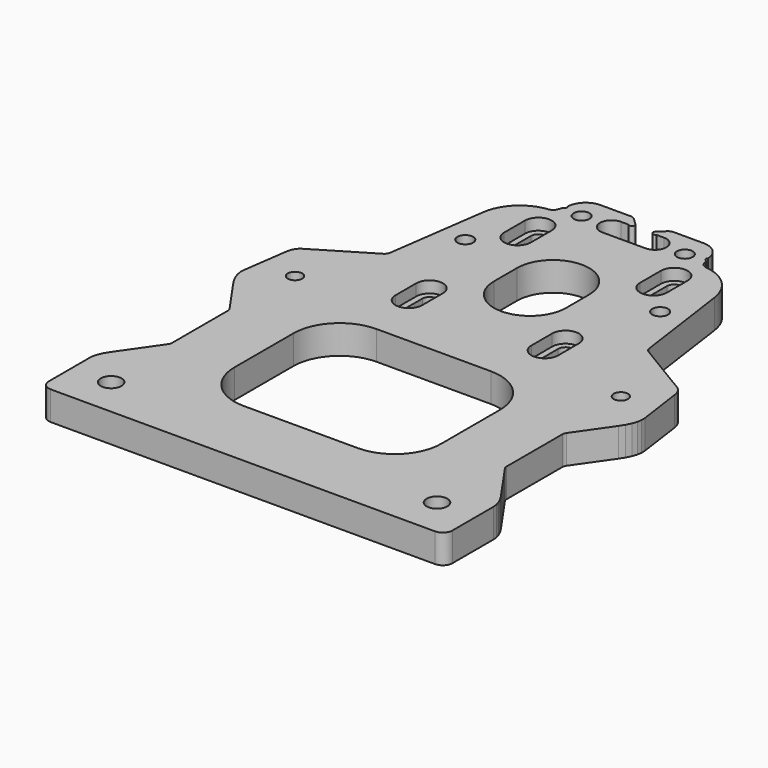
from build123d import *

# Parameters (mm, degrees)
F0_R     = 4.1
F0_R_2   = 2.725
F0_R_3   = 2.5
F0_R_4   = 3.6
F1_DEPTH = 10
F2_DEPTH = 6
F3_DEPTH = 4


# Not quite as in the source:
# - ends of sketch curves that miss each other by under 0.0002 mm in the source are joined


with BuildPart() as f1:
    # F0 (on Top) → F1 (new body)
    with BuildSketch(Plane.XY):
        with BuildLine():
            ThreePointArc((-70, -85.3407), (-69.01608381, -87.71608381), (-66.6407, -88.7))
            Line((-66.6407, -88.7), (66.64, -88.7))
            ThreePointArc((66.64, -88.7), (69.0158787848, -87.7158787848), (70, -85.34))
            Line((70, -85.34), (70, -67.5895))
            Line((70, -67.5895), (69.865948, -66.201885))
            Line((69.865948, -66.201885), (69.445962, -64.711612))
            Line((69.445962, -64.711612), (68.73318, -63.151071))
            Line((68.73318, -63.151071), (67.734412, -61.538447))
            Line((67.734412, -61.538447), (58.431324, -48.174831))
            ThreePointArc((58.431324, -48.174831), (58.1178035717, -47.5357835753), (58.01, -46.832182))
            Line((58.01, -46.832182), (58.01, -22.760348))
            ThreePointArc((58.01, -22.760348), (58.1179689174, -22.0562197272), (58.4319545741, -21.4167927032))
            Line((58.4319545741, -21.4167927032), (66.783489, -9.432068))
            Line((66.783489, -9.432068), (67.913719, -7.648339))
            Line((67.913719, -7.648339), (68.762828, -5.93532))
            Line((68.762828, -5.93532), (69.316332, -4.305329))
            Line((69.316332, -4.305329), (69.565046, -2.784029))
            Line((69.565046, -2.784029), (69.518711, -1.391715))
            Line((69.518711, -1.391715), (67.309142, 14.330181))
            Line((67.309142, 14.330181), (66.999212, 15.650057))
            Line((66.999212, 15.650057), (66.487155, 16.737863))
            Line((66.487155, 16.737863), (65.781814, 17.619854))
            Line((65.781814, 17.619854), (64.875084, 18.317561))
            Line((64.875084, 18.317561), (46.034788, 29.637953))
            ThreePointArc((46.034788, 29.637953), (45.2854954651, 30.3552438624), (44.917997067, 31.3252390094))
            Line((44.917997067, 31.3252390094), (40.093666, 65.65214))
            ThreePointArc((40.093666, 65.65214), (35.8358190199, 74.0012505725), (27.3375349502, 77.9529685197))
            ThreePointArc((27.3375349502, 77.9529685197), (26.1084756666, 78.4580664195), (25.3498539146, 79.5490309716))
            Line((25.3498539146, 79.5490309716), (24.828406, 81.117409))
            ThreePointArc((24.828406, 81.117409), (24.1173215696, 81.671357459), (24.355163875, 82.5408001437))
            ThreePointArc((24.355163875, 82.5408001437), (22.3679675258, 86.9125704183), (17.910791, 88.7))
            Line((17.910791, 88.7), (7.437437, 88.7))
            ThreePointArc((7.437437, 88.7), (6.5667217917, 88.5327402562), (5.8199517771, 88.0547702349))
            Line((5.8199517771, 88.0547702349), (3.5, 85.8536))
            ThreePointArc((3.5, 85.8536), (3.4660810953, 84.4733300764), (4.8463500657, 84.5072999404))
            Line((4.8463500657, 84.5072999404), (7.5, 84.5073))
            ThreePointArc((7.5, 84.5073), (11.5, 80.5073), (7.5, 76.5073))
            Line((7.5, 76.5073), (-7.5, 76.5073))
            ThreePointArc((-7.5, 76.5073), (-11.5, 80.5073), (-7.5, 84.5073))
            Line((-7.5, 84.5073), (-4.84635, 84.5073))
            ThreePointArc((-4.84635, 84.5073), (-3.4660810953, 84.4733300764), (-3.4999997219, 85.8536003068))
            Line((-3.4999997219, 85.8536003068), (-5.819951, 88.05477))
            ThreePointArc((-5.819951, 88.05477), (-6.5667214548, 88.5327401218), (-7.437437, 88.7))
            Line((-7.437437, 88.7), (-17.91079, 88.7))
            ThreePointArc((-17.91079, 88.7), (-22.3679665258, 86.9125704183), (-24.3551631887, 82.5408000085))
            ThreePointArc((-24.3551631887, 82.5408000085), (-24.1173207269, 81.6713569858), (-24.8284060254, 81.1174093435))
            Line((-24.8284060254, 81.1174093435), (-25.349853, 79.549031))
            ThreePointArc((-25.349853, 79.549031), (-26.1084746666, 78.4580664195), (-27.3375339495, 77.9529685125))
            ThreePointArc((-27.3375339495, 77.9529685125), (-35.8358186118, 74.001250966), (-40.0936657548, 65.6521401061))
            Line((-40.0936657548, 65.6521401061), (-44.917996, 31.325239))
            ThreePointArc((-44.917996, 31.325239), (-45.2854944651, 30.3552438624), (-46.0347868046, 29.6379526747))
            Line((-46.0347868046, 29.6379526747), (-64.875083, 18.317561))
            Line((-64.875083, 18.317561), (-65.764804, 17.636264))
            Line((-65.764804, 17.636264), (-66.464414, 16.773352))
            Line((-66.464414, 16.773352), (-66.99028, 15.673609))
            Line((-66.99028, 15.673609), (-67.30828, 14.330181))
            Line((-67.30828, 14.330181), (-69.517848, -1.391715))
            Line((-69.517848, -1.391715), (-69.564686, -2.784465))
            Line((-69.564686, -2.784465), (-69.316601, -4.307546))
            Line((-69.316601, -4.307546), (-68.763454, -5.938605))
            Line((-68.763454, -5.938605), (-67.915019, -7.650791))
            Line((-67.915019, -7.650791), (-66.786009, -9.432068))
            Line((-66.786009, -9.432068), (-58.427898, -21.419694))
            ThreePointArc((-58.427898, -21.419694), (-58.1136589115, -22.059327239), (-58.0056, -22.763742))
            Line((-58.0056, -22.763742), (-58.0056, -46.834916))
            ThreePointArc((-58.0056, -46.834916), (-58.1134934129, -47.5388038122), (-58.4272664273, -48.1780577023))
            Line((-58.4272664273, -48.1780577023), (-67.733176, -61.538447))
            Line((-67.733176, -61.538447), (-68.732469, -63.151034))
            Line((-68.732469, -63.151034), (-69.445644, -64.711573))
            Line((-69.445644, -64.711573), (-69.865872, -66.201869))
            Line((-69.865872, -66.201869), (-70, -67.5895))
            Line((-70, -67.5895), (-70, -85.3407))
        make_face()
        with Locations((-56.5, -75.18)):
            Circle(F0_R, mode=Mode.SUBTRACT)
        with Locations((56.5, -75.18)):
            Circle(F0_R, mode=Mode.SUBTRACT)
        with BuildLine():
            Line((19.8032, -63.6519), (-19.8032, -63.6519))
            ThreePointArc((-19.8032, -63.6519), (-31.1500010963, -58.9519010963), (-35.85, -47.6051))
            Line((-35.85, -47.6051), (-35.85, -21.9987))
            ThreePointArc((-35.85, -21.9987), (-31.1500010963, -10.6518989037), (-19.8032, -5.9519))
            Line((-19.8032, -5.9519), (19.8032, -5.9519))
            ThreePointArc((19.8032, -5.9519), (31.1500010963, -10.6518989037), (35.85, -21.9987))
            Line((35.85, -21.9987), (35.85, -47.6051))
            ThreePointArc((35.85, -47.6051), (31.1500010963, -58.9519010963), (19.8032, -63.6519))
        make_face(mode=Mode.SUBTRACT)
        with Locations((-56.5, 4.52)):
            Circle(F0_R, mode=Mode.SUBTRACT)
        with BuildLine():
            Line((-28.21, 12.7), (-28.21, 21.7))
            ThreePointArc((-28.21, 21.7), (-23.57, 26.34), (-18.93, 21.7))
            Line((-18.93, 21.7), (-18.93, 12.7))
            ThreePointArc((-18.93, 12.7), (-23.57, 8.06), (-28.21, 12.7))
        make_face(mode=Mode.SUBTRACT)
        with Locations((-33.8, 49.95)):
            Circle(F0_R_2, mode=Mode.SUBTRACT)
        with BuildLine():
            Line((-28.21, 59.84), (-28.21, 68.84))
            ThreePointArc((-28.21, 68.84), (-23.57, 73.48), (-18.93, 68.84))
            Line((-18.93, 68.84), (-18.93, 59.84))
            ThreePointArc((-18.93, 59.84), (-23.57, 55.2), (-28.21, 59.84))
        make_face(mode=Mode.SUBTRACT)
        with Locations((-17.9, 80.5073)):
            Circle(F0_R_2, mode=Mode.SUBTRACT)
        with BuildLine():
            Line((18.93, 12.7), (18.93, 21.7))
            ThreePointArc((18.93, 21.7), (23.57, 26.34), (28.21, 21.7))
            Line((28.21, 21.7), (28.21, 12.7))
            ThreePointArc((28.21, 12.7), (23.57, 8.06), (18.93, 12.7))
        make_face(mode=Mode.SUBTRACT)
        with BuildLine():
            Line((-12.5, 35.77), (-12.5, 45.77))
            ThreePointArc((-12.5, 45.77), (0, 58.27), (12.5, 45.77))
            Line((12.5, 45.77), (12.5, 35.77))
            ThreePointArc((12.5, 35.77), (0, 23.27), (-12.5, 35.77))
        make_face(mode=Mode.SUBTRACT)
        with Locations((56.5, 4.52)):
            Circle(F0_R, mode=Mode.SUBTRACT)
        with Locations((33.8, 49.95)):
            Circle(F0_R_2, mode=Mode.SUBTRACT)
        with BuildLine():
            Line((18.93, 59.84), (18.93, 68.84))
            ThreePointArc((18.93, 68.84), (23.57, 73.48), (28.21, 68.84))
            Line((28.21, 68.84), (28.21, 59.84))
            ThreePointArc((28.21, 59.84), (23.57, 55.2), (18.93, 59.84))
        make_face(mode=Mode.SUBTRACT)
        with Locations((17.9, 80.5073)):
            Circle(F0_R_2, mode=Mode.SUBTRACT)
        with Locations((-56.5, 4.52)):
            Circle(F0_R)
        with Locations((-56.5, 4.52)):
            Circle(F0_R_3, mode=Mode.SUBTRACT)
        with Locations((56.5, 4.52)):
            Circle(F0_R)
        with Locations((56.5, 4.52)):
            Circle(F0_R_3, mode=Mode.SUBTRACT)
        with Locations((56.5, -75.18)):
            Circle(F0_R)
        with Locations((56.5, -75.18)):
            Circle(F0_R_4, mode=Mode.SUBTRACT)
        with Locations((-56.5, -75.18)):
            Circle(F0_R)
        with Locations((-56.5, -75.18)):
            Circle(F0_R_4, mode=Mode.SUBTRACT)
    extrude(amount=F1_DEPTH)

    # F0 (on Top) → F2 (join)
    with BuildSketch(Plane.XY):
        with BuildLine():
            ThreePointArc((-18.93, 21.7), (-23.57, 26.34), (-28.21, 21.7))
            Line((-28.21, 21.7), (-28.21, 12.7))
            ThreePointArc((-28.21, 12.7), (-23.57, 8.06), (-18.93, 12.7))
            Line((-18.93, 12.7), (-18.93, 21.7))
        make_face()
        with BuildLine():
            Line((-26.11, 12.7), (-26.11, 21.7))
            ThreePointArc((-26.11, 21.7), (-23.57, 24.24), (-21.03, 21.7))
            Line((-21.03, 21.7), (-21.03, 12.7))
            ThreePointArc((-21.03, 12.7), (-23.57, 10.16), (-26.11, 12.7))
        make_face(mode=Mode.SUBTRACT)
        with BuildLine():
            ThreePointArc((-18.93, 68.84), (-23.57, 73.48), (-28.21, 68.84))
            Line((-28.21, 68.84), (-28.21, 59.84))
            ThreePointArc((-28.21, 59.84), (-23.57, 55.2), (-18.93, 59.84))
            Line((-18.93, 59.84), (-18.93, 68.84))
        make_face()
        with BuildLine():
            Line((-26.11, 59.84), (-26.11, 68.84))
            ThreePointArc((-26.11, 68.84), (-23.57, 71.38), (-21.03, 68.84))
            Line((-21.03, 68.84), (-21.03, 59.84))
            ThreePointArc((-21.03, 59.84), (-23.57, 57.3), (-26.11, 59.84))
        make_face(mode=Mode.SUBTRACT)
        with BuildLine():
            ThreePointArc((28.21, 68.84), (23.57, 73.48), (18.93, 68.84))
            Line((18.93, 68.84), (18.93, 59.84))
            ThreePointArc((18.93, 59.84), (23.57, 55.2), (28.21, 59.84))
            Line((28.21, 59.84), (28.21, 68.84))
        make_face()
        with BuildLine():
            Line((21.03, 59.84), (21.03, 68.84))
            ThreePointArc((21.03, 68.84), (23.57, 71.38), (26.11, 68.84))
            Line((26.11, 68.84), (26.11, 59.84))
            ThreePointArc((26.11, 59.84), (23.57, 57.3), (21.03, 59.84))
        make_face(mode=Mode.SUBTRACT)
        with BuildLine():
            ThreePointArc((28.21, 21.7), (23.57, 26.34), (18.93, 21.7))
            Line((18.93, 21.7), (18.93, 12.7))
            ThreePointArc((18.93, 12.7), (23.57, 8.06), (28.21, 12.7))
            Line((28.21, 12.7), (28.21, 21.7))
        make_face()
        with BuildLine():
            Line((21.03, 12.7), (21.03, 21.7))
            ThreePointArc((21.03, 21.7), (23.57, 24.24), (26.11, 21.7))
            Line((26.11, 21.7), (26.11, 12.7))
            ThreePointArc((26.11, 12.7), (23.57, 10.16), (21.03, 12.7))
        make_face(mode=Mode.SUBTRACT)
    extrude(amount=F2_DEPTH)

    # F0 (on Top) → F3 (cut, through all)
    with BuildSketch(Plane.XY):
        with Locations((-56.5, -75.18)):
            Circle(F0_R)
        with Locations((-56.5, -75.18)):
            Circle(F0_R_4, mode=Mode.SUBTRACT)
        with Locations((-56.5, 4.52)):
            Circle(F0_R)
        with Locations((-56.5, 4.52)):
            Circle(F0_R_3, mode=Mode.SUBTRACT)
        with Locations((56.5, 4.52)):
            Circle(F0_R)
        with Locations((56.5, 4.52)):
            Circle(F0_R_3, mode=Mode.SUBTRACT)
        with Locations((56.5, -75.18)):
            Circle(F0_R)
        with Locations((56.5, -75.18)):
            Circle(F0_R_4, mode=Mode.SUBTRACT)
    extrude(amount=F3_DEPTH, mode=Mode.SUBTRACT)


solid = f1.part
